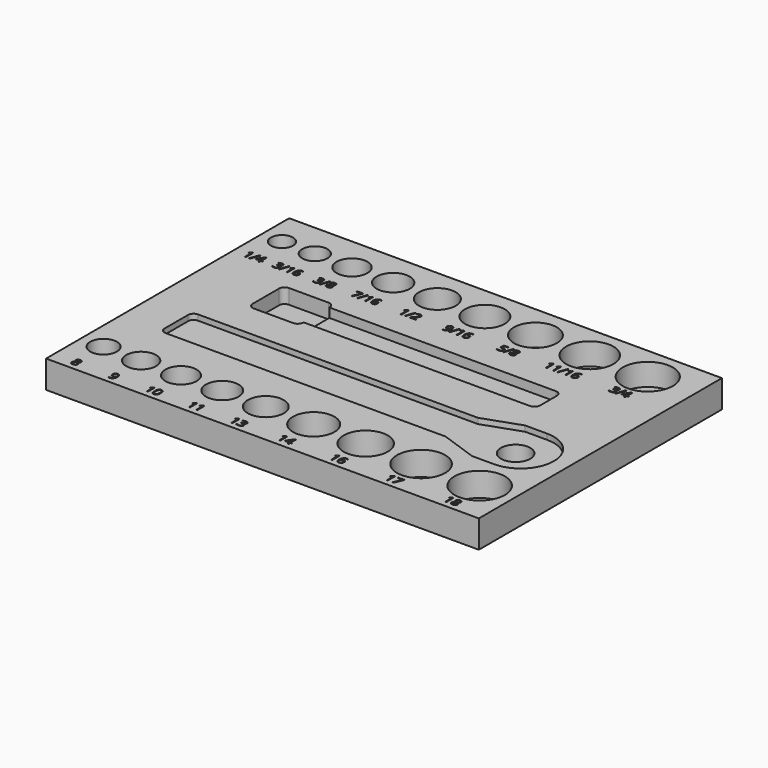
from build123d import *

# Parameters (mm, degrees)
F0_W          = 235
F0_H          = 165
F1_DEPTH      = 15
F2_R          = 7.25
F2_R_2        = 13.7
F2_R_3        = 13.1
F2_R_4        = 12
F2_R_5        = 11.25
F2_R_6        = 9.75
F2_R_7        = 8.9
F2_R_8        = 8.5
F2_R_9        = 8.15
F3_DEPTH      = 13
F5_TEXT_SIZE  = 6.9444444444
F6_DEPTH      = 1
F7_R          = 7.25
F7_R_2        = 8
F8_DEPTH      = 3
F9_R          = 8
F10_DEPTH     = 25
F12_DEPTH     = 5
F13_R         = 6
F13_R_2       = 6.85
F13_R_3       = 8.35
F13_R_4       = 9
F13_R_5       = 10
F13_R_6       = 10.8
F13_R_7       = 11.65
F13_R_8       = 12.85
F13_R_9       = 13.65
F14_DEPTH     = 12
F15_TEXT_SIZE = 6.9444444444
F16_DEPTH     = 1
F18_DEPTH     = 8


# Not quite as in the source:
# - Text() gives the source's letters only with a copy of the font that has no kerning and outlines rounded to 1/6400 em; it was checked with that copy


with BuildPart() as f1:
    # F0 (on Top) → F1 (new body)
    with BuildSketch(Plane.XY):
        with Locations((117.5, 82.5)):
            Rectangle(F0_W, F0_H)
    extrude(amount=F1_DEPTH)

    # F2 (on face) → F3 (cut)
    with BuildSketch(Plane.XY.offset(15)):
        with Locations((12.25, 23.7)):
            Circle(F2_R)
        with Locations((216.5, 23.7)):
            Circle(F2_R_2)
        with Locations((184.7, 23.7)):
            Circle(F2_R_3)
        with Locations((154.6, 23.7)):
            Circle(F2_R_4)
        with Locations((126.35, 23.7)):
            Circle(F2_R_5)
        with Locations((100.35, 23.7)):
            Circle(F2_R_6)
        with Locations((76.7, 23.7)):
            Circle(F2_R_7)
        with Locations((54.3, 23.7)):
            Circle(F2_R_8)
        with Locations((32.65, 23.7)):
            Circle(F2_R_9)
    extrude(amount=-F3_DEPTH, mode=Mode.SUBTRACT)

    # F5 (on face) → F6 (cut)
    with BuildSketch(Plane.XY.offset(15)):
        with Locations((10.2192925347, 3)):
            Text('8', F5_TEXT_SIZE, font='Open Sans', text_align=(TextAlign.LEFT, TextAlign.BOTTOM))
        with Locations((30.6258029514, 3)):
            Text('9', F5_TEXT_SIZE, font='Open Sans', text_align=(TextAlign.LEFT, TextAlign.BOTTOM))
        with Locations((50.2771050347, 3)):
            Text('10', F5_TEXT_SIZE, font='Open Sans', text_align=(TextAlign.LEFT, TextAlign.BOTTOM))
        with Locations((73.2776909722, 3)):
            Text('11', F5_TEXT_SIZE, font='Open Sans', text_align=(TextAlign.LEFT, TextAlign.BOTTOM))
        with Locations((96.3580295139, 3)):
            Text('13', F5_TEXT_SIZE, font='Open Sans', text_align=(TextAlign.LEFT, TextAlign.BOTTOM))
        with Locations((122.2240234375, 3)):
            Text('14', F5_TEXT_SIZE, font='Open Sans', text_align=(TextAlign.LEFT, TextAlign.BOTTOM))
        with Locations((150.5738498264, 3)):
            Text('16', F5_TEXT_SIZE, font='Open Sans', text_align=(TextAlign.LEFT, TextAlign.BOTTOM))
        with Locations((180.6809027778, 3)):
            Text('17', F5_TEXT_SIZE, font='Open Sans', text_align=(TextAlign.LEFT, TextAlign.BOTTOM))
        with Locations((212.4841579861, 3)):
            Text('18', F5_TEXT_SIZE, font='Open Sans', text_align=(TextAlign.LEFT, TextAlign.BOTTOM))
    extrude(amount=-F6_DEPTH, mode=Mode.SUBTRACT)

    # F7 (on face) → F8 (cut)
    with BuildSketch(Plane.XY.offset(15)):
        with Locations((12.25, 23.7)):
            Circle(F7_R)
        with BuildLine():
            Line((85, 71.9), (25, 71.9))
            ThreePointArc((25, 71.9), (22.8786796564, 71.0213203436), (22, 68.9))
            Line((22, 68.9), (22, 60.9))
            Line((22, 60.9), (22, 52.9))
            ThreePointArc((22, 52.9), (22.8786796564, 50.7786796564), (25, 49.9))
            Line((25, 49.9), (177, 49.9))
            Line((177, 49.9), (197, 42.9))
            Line((197, 42.9), (209, 42.9))
            ThreePointArc((209, 42.9), (221.7279220614, 48.1720779386), (227, 60.9))
            ThreePointArc((227, 60.9), (221.7279220614, 73.6279220614), (209, 78.9))
            Line((209, 78.9), (197, 78.9))
            Line((197, 78.9), (177, 71.9))
            Line((177, 71.9), (135, 71.9))
            Line((135, 71.9), (85, 71.9))
        make_face()
        with Locations((206.25, 60.9)):
            Circle(F7_R_2, mode=Mode.SUBTRACT)
    extrude(amount=-F8_DEPTH, mode=Mode.SUBTRACT)

    # F9 (on face) → F10 (cut)
    with BuildSketch(Plane.XY.offset(15)):
        with Locations((206.25, 60.9)):
            Circle(F9_R)
    extrude(amount=-F10_DEPTH, mode=Mode.SUBTRACT)

    # F11 (on face) → F12 (cut)
    with BuildSketch(Plane.XY.offset(15)):
        with BuildLine():
            Line((61.5, 114.9), (40, 114.9))
            ThreePointArc((40, 114.9), (37.8786796564, 114.0213203436), (37, 111.9))
            Line((37, 111.9), (37, 102.9))
            Line((37, 102.9), (37, 93.9))
            ThreePointArc((37, 93.9), (37.8786796564, 91.7786796564), (40, 90.9))
            Line((40, 90.9), (61.5, 90.9))
            ThreePointArc((61.5, 90.9), (63.6213203436, 91.7786796564), (64.5, 93.9))
            Line((64.5, 93.9), (64.5, 94.15))
            Line((64.5, 94.15), (187.5, 94.15))
            ThreePointArc((187.5, 94.15), (189.6213203436, 95.0286796564), (190.5, 97.15))
            Line((190.5, 97.15), (190.5, 102.9))
            Line((190.5, 102.9), (190.5, 108.65))
            ThreePointArc((190.5, 108.65), (189.6213203436, 110.7713203436), (187.5, 111.65))
            Line((187.5, 111.65), (64.5, 111.65))
            Line((64.5, 111.65), (64.5, 111.9))
            ThreePointArc((64.5, 111.9), (63.6213203436, 114.0213203436), (61.5, 114.9))
        make_face()
    extrude(amount=-F12_DEPTH, mode=Mode.SUBTRACT)

    # F13 (on face) → F14 (cut)
    with BuildSketch(Plane.XY.offset(15)):
        with Locations((11, 146.35)):
            Circle(F13_R)
        with Locations((28.85, 146.35)):
            Circle(F13_R_2)
        with Locations((49.05, 146.35)):
            Circle(F13_R_3)
        with Locations((71.4, 146.35)):
            Circle(F13_R_4)
        with Locations((95.4, 146.35)):
            Circle(F13_R_5)
        with Locations((121.2, 146.35)):
            Circle(F13_R_6)
        with Locations((148.65, 146.35)):
            Circle(F13_R_7)
        with Locations((178.15, 146.35)):
            Circle(F13_R_8)
        with Locations((209.65, 146.35)):
            Circle(F13_R_9)
    extrude(amount=-F14_DEPTH, mode=Mode.SUBTRACT)

    # F15 (on face) → F16 (cut)
    with BuildSketch(Plane.XY.offset(15)):
        with Locations((5.5990668403, 125.7)):
            Text('1/4', F15_TEXT_SIZE, font='Open Sans', text_align=(TextAlign.LEFT, TextAlign.BOTTOM))
        with Locations((21.5637586806, 125.7)):
            Text('3/16', F15_TEXT_SIZE, font='Open Sans', text_align=(TextAlign.LEFT, TextAlign.BOTTOM))
        with Locations((43.7592013889, 125.7)):
            Text('3/8', F15_TEXT_SIZE, font='Open Sans', text_align=(TextAlign.LEFT, TextAlign.BOTTOM))
        with Locations((64.1137586806, 125.7)):
            Text('7/16', F15_TEXT_SIZE, font='Open Sans', text_align=(TextAlign.LEFT, TextAlign.BOTTOM))
        with Locations((90.1157118056, 125.7)):
            Text('1/2', F15_TEXT_SIZE, font='Open Sans', text_align=(TextAlign.LEFT, TextAlign.BOTTOM))
        with Locations((113.9137586806, 125.7)):
            Text('9/16', F15_TEXT_SIZE, font='Open Sans', text_align=(TextAlign.LEFT, TextAlign.BOTTOM))
        with Locations((143.3592013889, 125.7)):
            Text('5/8', F15_TEXT_SIZE, font='Open Sans', text_align=(TextAlign.LEFT, TextAlign.BOTTOM))
        with Locations((168.8786241319, 125.7)):
            Text('11/16', F15_TEXT_SIZE, font='Open Sans', text_align=(TextAlign.LEFT, TextAlign.BOTTOM))
        with Locations((204.2490668403, 125.7)):
            Text('3/4', F15_TEXT_SIZE, font='Open Sans', text_align=(TextAlign.LEFT, TextAlign.BOTTOM))
    extrude(amount=-F16_DEPTH, mode=Mode.SUBTRACT)

    # F17 (on face) → F18 (cut)
    with BuildSketch(Plane.XY.offset(15)):
        with BuildLine():
            Line((61.5, 114.9), (40, 114.9))
            ThreePointArc((40, 114.9), (37.8786796564, 114.0213203436), (37, 111.9))
            Line((37, 111.9), (37, 93.9))
            ThreePointArc((37, 93.9), (37.8786796564, 91.7786796564), (40, 90.9))
            Line((40, 90.9), (61.5, 90.9))
            ThreePointArc((61.5, 90.9), (63.6213203436, 91.7786796564), (64.5, 93.9))
            Line((64.5, 93.9), (64.5, 94.15))
            Line((64.5, 94.15), (64.5, 111.65))
            Line((64.5, 111.65), (64.5, 111.9))
            ThreePointArc((64.5, 111.9), (63.6213203436, 114.0213203436), (61.5, 114.9))
        make_face()
    extrude(amount=-F18_DEPTH, mode=Mode.SUBTRACT)


solid = f1.part
